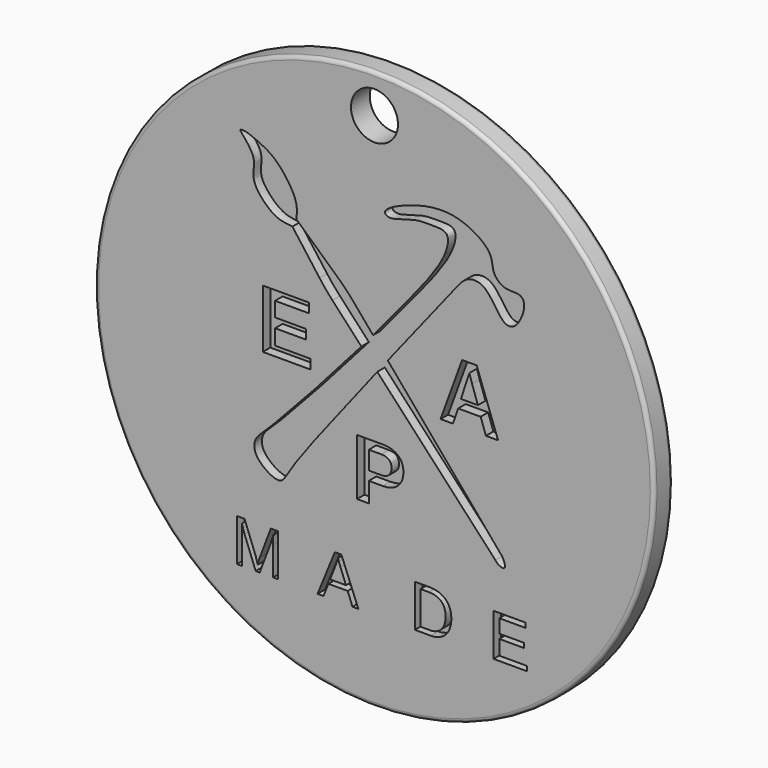
from build123d import *

# Parameters (mm, degrees)
F0_R           = 37.780695212
F2_DEPTH       = 3.175
F3_DEPTH       = 1.27
F5_DEPTH       = 1.27
F6_TEXT_SIZE   = 11.5909102735
F6_TEXT_SIZE_2 = 11.0878544446
F6_TEXT_SIZE_3 = 11.4809032918
F7_DEPTH       = 1.27
F8_TEXT_SIZE   = 8.3190802899
F9_DEPTH       = 1.27
F10_R          = 3.175
F11_DEPTH      = 3.176
F12_R          = 0.508
F13_SCALE      = 0.3333333333


# Not quite as in the source:
# - Text() gives the source's letters only with a copy of the font that has no kerning and outlines rounded to 1/6400 em; it was checked with that copy


with BuildPart() as f2:
    # F0 (on Front) → F2 (new body)
    with BuildSketch(Plane.XZ):
        with Locations((0, -4.1949953884)):
            Circle(F0_R)
    extrude(amount=-F2_DEPTH)

    # F1 (on Front) → F3 (cut)
    with BuildSketch(Plane.XZ):
        with BuildLine():
            add(Edge.make_bspline(
                [(9.415787092, 14.7911859462), (8.5089660445, 12.7604264422), (4.1731654019, 7.4183880177), (-3.592955155, -1.9920661215), (-14.4019461802, -13.7469650283), (-16.2315302796, -15.1816178262), (-16.397118169, -17.5648206434), (-12.6947389795, -19.9251287459), (-11.5433806926, -17.3772387896), (-4.5728139741, -8.185447484), (10.3678865747, 10.6750395007), (12.4583515626, 13.3049864039), (15.2937603761, 13.2041495797), (17.1446661515, 9.1331036507), (18.9043245728, 9.210140236), (19.8355663216, 10.5561863157), (20.4634734471, 12.4922458304), (19.6974644843, 13.6912469506), (17.5175937114, 13.2634329714), (15.7912677456, 14.944519869), (16.1312628433, 17.3180620197), (11.3530086664, 20.4950062472), (5.7711532121, 19.8914368339), (1.3843008673, 17.9220379849), (1.396853445, 17.0618404278), (2.4293533792, 16.6969652239), (5.4201638764, 17.9460510939), (7.7225360316, 17.8309290186), (10.2874482772, 17.8741127994), (9.9311453034, 15.9452930202), (9.415787092, 14.7911859462)],
                knots=[0, 0, 0, 0, 0.0534884757, 0.1220878558, 0.1948932693, 0.2213529565, 0.2470821615, 0.2817112027, 0.3060680604, 0.3704654363, 0.4623053487, 0.4939632429, 0.521100557, 0.5586132346, 0.5795638688, 0.602651635, 0.6286607917, 0.6478196121, 0.6739151715, 0.7004005782, 0.7269185319, 0.768104569, 0.8137001334, 0.8521931143, 0.8649043541, 0.881846698, 0.9147657156, 0.9443761259, 0.9696018026, 1, 1, 1, 1], degree=3))
        make_face()
    extrude(amount=-F3_DEPTH, mode=Mode.SUBTRACT)

    # F4 (on Front) → F5 (cut)
    with BuildSketch(Plane.XZ):
        with BuildLine():
            Line((-5.0839400313, 7.6377649066), (-10.5388658121, 12.5971781427))
            add(Edge.make_bspline(
                [(-10.5388658121, 12.5971781427), (-10.4717037736, 13.1895145383), (-10.3879902506, 14.3896601716), (-11.3218707691, 16.4104971781), (-13.2508589508, 18.868941504), (-15.1734568199, 19.9877163076), (-17.5054007451, 20.9703747276), (-18.2624626815, 20.8037821465), (-17.7514585787, 20.2872338103), (-16.1895923209, 18.3756284167), (-16.3068753823, 16.9059177345), (-16.4564560182, 15.2601548802), (-15.2575521624, 13.5185772704), (-13.297555422, 11.7774268673), (-11.8114249137, 11.6478519227), (-11.0862655565, 11.5667367354)],
                knots=[0, 0, 0, 0, 0.0749814908, 0.1592301565, 0.2587423851, 0.346734382, 0.4365547706, 0.4751755944, 0.5150213017, 0.6041236137, 0.6732344231, 0.7436577642, 0.8252487617, 0.9162202808, 1, 1, 1, 1], degree=3))
            Line((-11.0862655565, 11.5667367354), (-7.4173012051, 6.6436512654))
            ThreePointArc((-7.4173012051, 6.6436512654), (-6.5741271483, 5.5734164879), (-5.6747784927, 4.5499337256))
            Line((-5.6747784927, 4.5499337256), (16.3364037871, -19.1841367632))
            add(Edge.make_bspline(
                [(17.2721613199, -18.4729620814), (17.396526246, -18.7388130833), (17.6707884426, -19.1909917385), (17.6191879339, -19.974562763), (16.6934698581, -19.6223353537), (16.440516284, -19.330107043), (16.3364037871, -19.1841367632)],
                knots=[0, 0, 0, 0, 0.2819569505, 0.5015186489, 0.7663662806, 1, 1, 1, 1], degree=3))
            Line((17.2721613199, -18.4729620814), (-2.771959826, 5.2407279098))
            ThreePointArc((-2.771959826, 5.2407279098), (-3.8886216873, 6.4771791208), (-5.0839400313, 7.6377649066))
        make_face()
    extrude(amount=-F5_DEPTH, mode=Mode.SUBTRACT)

    # F6 (on face) → F7 (cut)
    with BuildSketch(Plane.XZ):
        with Locations((8.6426539347, -4.8206776846)):
            Text('A', F6_TEXT_SIZE, font='Arimo', font_style=FontStyle.BOLD, text_align=(TextAlign.LEFT, TextAlign.BOTTOM))
        with Locations((-3.1062052585, -18.0054698139)):
            Text('P', F6_TEXT_SIZE_2, font='Arimo', font_style=FontStyle.BOLD, text_align=(TextAlign.LEFT, TextAlign.BOTTOM))
        with Locations((-15.855897218, -4.6423131134)):
            Text('E', F6_TEXT_SIZE_3, font='Arimo', font_style=FontStyle.BOLD, text_align=(TextAlign.LEFT, TextAlign.BOTTOM))
    extrude(amount=-F7_DEPTH, mode=Mode.SUBTRACT)

    # F8 (on face) → F9 (cut)
    with BuildSketch(Plane.XZ):
        with Locations((-19.2587822676, -31.0191251338)):
            Text('M  A   D  E', F8_TEXT_SIZE, font='Arimo', text_align=(TextAlign.LEFT, TextAlign.BOTTOM))
    extrude(amount=-F9_DEPTH, mode=Mode.SUBTRACT)

    # F10 (on face) → F11 (cut, through all)
    with BuildSketch(Plane.XZ):
        with Locations((0, 28.3632650971)):
            Circle(F10_R)
    extrude(amount=-F11_DEPTH, mode=Mode.SUBTRACT)

    # F12
    f12_edges = [f2.edges().sort_by_distance(p)[0] for p in [
        (-37.780695, 0, -4.194995),
        (-37.780695, 3.175, -4.194995),
    ]]
    fillet(f12_edges, radius=F12_R)


with BuildPart() as f2_1:
    # F13: moved
    add(f2.part.scale(F13_SCALE))


solid = f2_1.part
